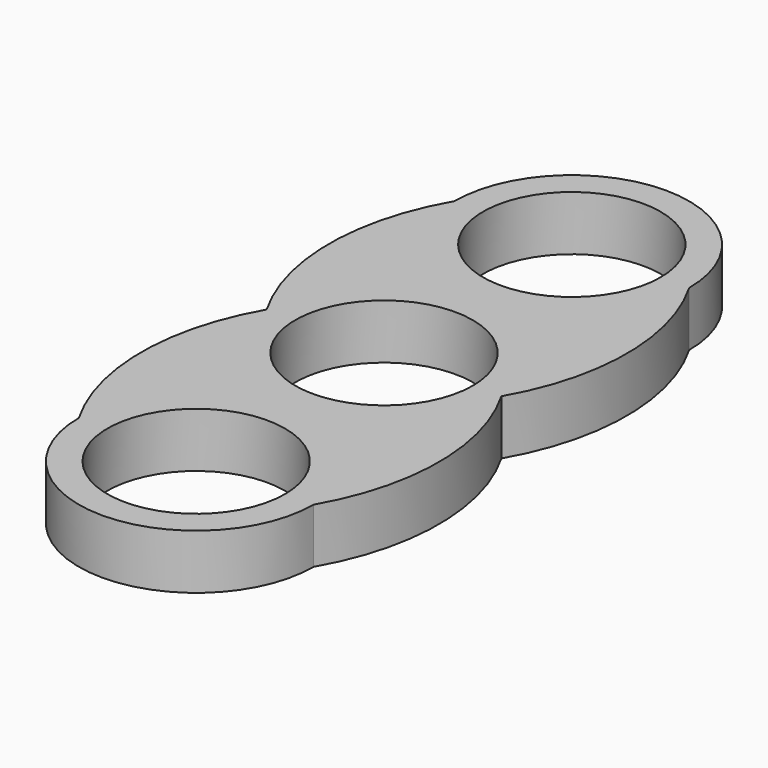
from build123d import *

# Parameters (mm, degrees)
F0_R     = 11.35
F1_DEPTH = 7


# Not quite as in the source:
# - a feature names something its author has since deleted; it is built from what else it names


with BuildPart() as f1:
    # F0 (on Top) → F1 (new body)
    with BuildSketch(Plane.XY):
        with BuildLine():
            ThreePointArc((0, -15), (10.6066017178, -10.6066017178), (15, 0))
            ThreePointArc((15, 0), (10.6066016959, 10.6066017397), (-6.18e-08, 15))
            ThreePointArc((-6.18e-08, 15), (-10.6066017397, 10.6066016959), (-15, 0))
            ThreePointArc((-15, 0), (-10.6066017178, -10.6066017178), (0, -15))
        make_face()
        Circle(F0_R, mode=Mode.SUBTRACT)
        with BuildLine():
            ThreePointArc((15, -30), (19.0192378865, -15), (15, 0))
            ThreePointArc((15, 0), (10.6066017178, -10.6066017178), (0, -15))
            ThreePointArc((0, -15), (10.6066017178, -19.3933982822), (15, -30))
        make_face()
        with BuildLine():
            ThreePointArc((-6.18e-08, 15), (10.6066016959, 10.6066017397), (15, 0))
            ThreePointArc((15, 0), (19.0192378865, 15), (15, 30))
            ThreePointArc((15, 30), (10.6066016959, 19.3933982603), (-6.18e-08, 15))
        make_face()
        with BuildLine():
            ThreePointArc((-15, 0), (-10.6066017397, 10.6066016959), (-6.18e-08, 15))
            ThreePointArc((-6.18e-08, 15), (-10.6066017397, 19.3933983041), (-15, 30))
            ThreePointArc((-15, 30), (-19.0192378865, 15), (-15, 0))
        make_face()
        with BuildLine():
            ThreePointArc((-15, 30), (-10.6066017397, 19.3933983041), (-6.18e-08, 15))
            ThreePointArc((-6.18e-08, 15), (10.6066016959, 19.3933982603), (15, 30))
            ThreePointArc((15, 30), (0, 45), (-15, 30))
        make_face()
        with Locations((0, 30)):
            Circle(F0_R, mode=Mode.SUBTRACT)
        with BuildLine():
            ThreePointArc((-15, -30), (-10.6066017178, -19.3933982822), (0, -15))
            ThreePointArc((0, -15), (-10.6066017178, -10.6066017178), (-15, 0))
            ThreePointArc((-15, 0), (-19.0192378865, -15), (-15, -30))
        make_face()
        with BuildLine():
            ThreePointArc((15, -30), (10.6066017178, -19.3933982822), (0, -15))
            ThreePointArc((0, -15), (-10.6066017178, -19.3933982822), (-15, -30))
            ThreePointArc((-15, -30), (0, -45), (15, -30))
        make_face()
        with Locations((0, -30)):
            Circle(F0_R, mode=Mode.SUBTRACT)
    extrude(amount=F1_DEPTH)


solid = f1.part
